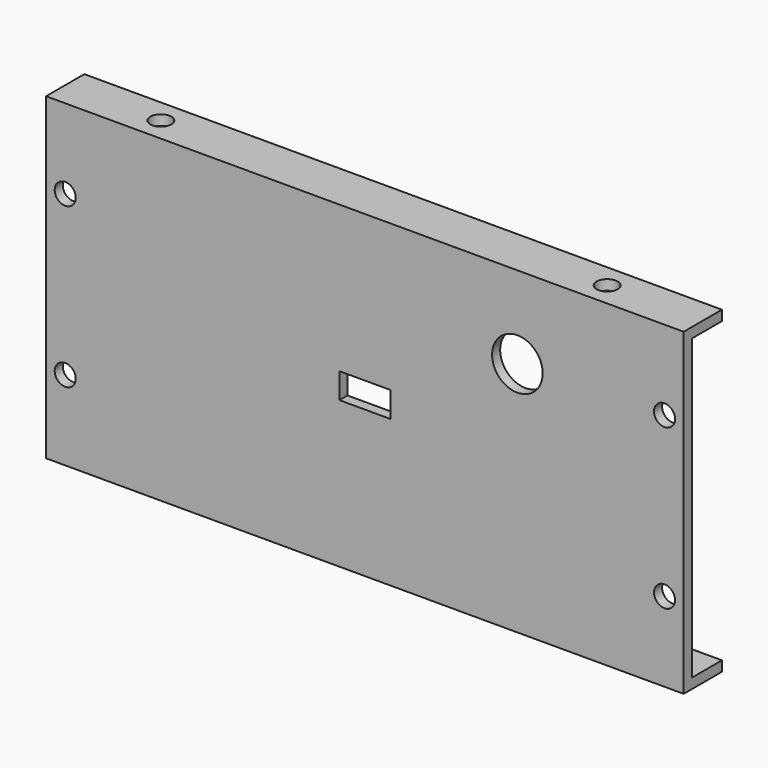
from build123d import *

# Parameters (mm, degrees)
F1_DEPTH      = 100
F2_W          = 16
F2_H          = 8
F2_R          = 3.3
F3_DEPTH      = 228
F3_DEPTH_BACK = 15.001
F4_R          = 3.3
F5_DEPTH      = 100.001
F6_R          = 7.9375
F7_DEPTH      = 15.001


# Not quite as in the source:
# - an extrude ends at something that could not be found from the text; its depth is read off the source's solid


with BuildPart() as f1:
    # F0 (on Right) → F1 (new body, symmetric)
    with BuildSketch(Plane.YZ):
        Polygon((13.4125, 50), (1.5875, 50), (-1.5875, 50), (-1.5875, 46.825), (-1.5875, -46.825), (-1.5875, -50), (1.5875, -50), (13.4125, -50), (13.4125, -46.825), (1.5875, -46.825), (1.5875, 46.825), (13.4125, 46.825), align=None)
    extrude(amount=F1_DEPTH, both=True)

    # F2 (on face) → F3 (cut, two sides)
    with BuildSketch(Plane.XZ.offset(1.5875)) as f3_sk:
        Rectangle(F2_W, F2_H)
        with Locations((94, -25)):
            Circle(F2_R)
        with Locations((94, 25)):
            Circle(F2_R)
        with Locations((-94, -25)):
            Circle(F2_R)
        with Locations((-94, 25)):
            Circle(F2_R)
    extrude(amount=F3_DEPTH, mode=Mode.SUBTRACT)
    extrude(f3_sk.sketch, amount=-F3_DEPTH_BACK, mode=Mode.SUBTRACT)

    # F4 (on face) → F5 (cut, through all)
    with BuildSketch(Plane.XY.offset(50)):
        with Locations((-70, 5.9125)):
            Circle(F4_R)
        with Locations((70, 5.9125)):
            Circle(F4_R)
    extrude(amount=-F5_DEPTH, mode=Mode.SUBTRACT)

    # F6 (on face) → F7 (cut, through all)
    with BuildSketch(Plane.XZ.offset(1.5875)):
        with Locations((47.8418069781, 24.1387402225)):
            Circle(F6_R)
    extrude(amount=-F7_DEPTH, mode=Mode.SUBTRACT)


solid = f1.part
